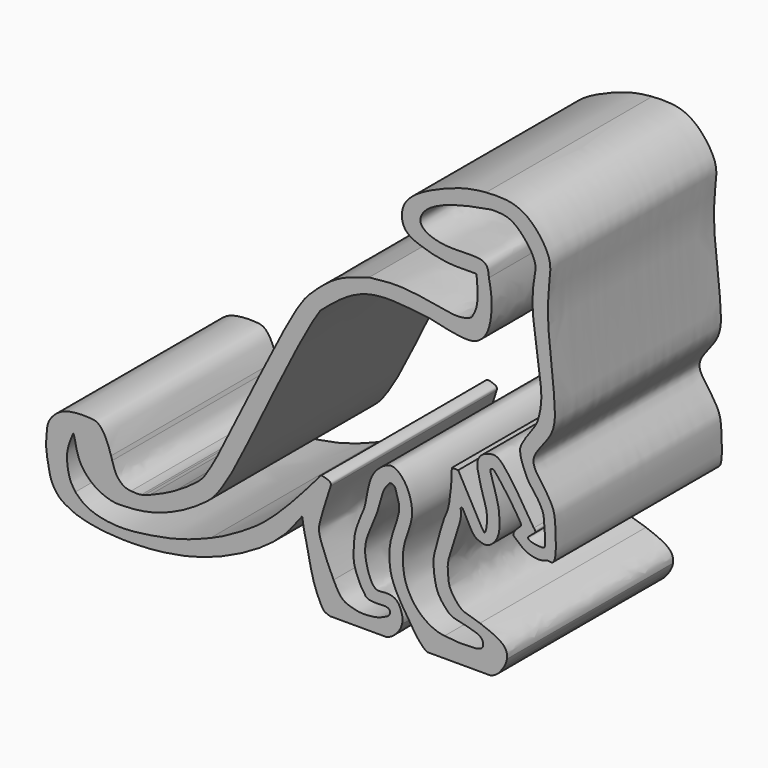
from build123d import *

# Parameters (mm, degrees)
F1_DEPTH = 15


with BuildPart() as f1:
    # F0 (on Front) → F1 (new body)
    with BuildSketch(Plane.XZ):
        with BuildLine():
            add(Edge.make_bspline(
                [(-15.4669350013, 23.1157913804), (-15.054879923, 23.1634013305), (-14.16984314, 23.2656608566), (-12.6167482466, 23.302404707), (-9.8137005936, 22.7928433269), (-8.9715752348, 22.6811060896), (-8.2451566536, 22.8389594973), (-8.03832151, 23.0131447315)],
                knots=[0, 0, 0, 0, 0.1348135249, 0.2895606307, 0.4912986818, 0.6066635572, 0.7214824154, 0.7214824154, 0.7214824154, 0.7214824154], degree=3))
            add(Edge.make_bspline(
                [(-15.4669350013, 23.1157913804), (-15.9986056397, 22.9585360257), (-17.0288350347, 22.6538187907), (-18.2910607324, 22.0040531604), (-19.6510649855, 20.7862506259), (-20.9749613494, 19.4248391371), (-26.1462638175, 8.5567205501), (-26.9967502917, 7.1942661965), (-27.6110490739, 6.1296289203), (-28.892969563, 5.3378997194), (-29.5255687088, 4.9558193423)],
                knots=[0, 0, 0, 0, 0.0832929576, 0.1614853434, 0.2445033573, 0.340585603, 0.5660088679, 0.6516770772, 0.7191066421, 0.8171798068, 0.8171798068, 0.8171798068, 0.8171798068], degree=3))
            add(Edge.make_bspline(
                [(-29.5255687088, 4.9558193423), (-30.0858358851, 4.6174263877), (-30.5959965363, 4.3182898855), (-31.2344844186, 4.148363515), (-31.2975818668, 4.1329435699)],
                knots=[0.8171798068, 0.8171798068, 0.8171798068, 0.8171798068, 0.9040391955, 0.9133811708, 0.9133811708, 0.9133811708, 0.9133811708], degree=3))
            add(Edge.make_bspline(
                [(-31.2975818668, 4.1329435699), (-31.4285690738, 4.083667204), (-31.5610759025, 4.0392471707), (-31.6864065826, 4.0075839497)],
                knots=[0.3472661829, 0.3472661829, 0.3472661829, 0.3472661829, 0.4123145482, 0.4123145482, 0.4123145482, 0.4123145482], degree=3))
            add(Edge.make_bspline(
                [(-31.9234459559, 3.935665863), (-31.8432725115, 3.9586455929), (-31.7648395471, 3.9831147713), (-31.6864065826, 4.0075839497)],
                knots=[0.9780776817, 0.9780776817, 0.9780776817, 0.9780776817, 1, 1, 1, 1], degree=3))
            add(Edge.make_bspline(
                [(-33.2431405897, 3.873629757), (-32.9938222307, 3.7955130583), (-32.4731148481, 3.7955338323), (-32.0677881033, 3.8942937655), (-31.9234459559, 3.935665863)],
                knots=[0.8714155003, 0.8714155003, 0.8714155003, 0.8714155003, 0.9386093201, 0.9780776817, 0.9780776817, 0.9780776817, 0.9780776817], degree=3))
            add(Edge.make_bspline(
                [(-38.7925319374, 5.3414250724), (-38.721084696, 5.9435743843), (-38.1788535617, 7.0706106992), (-36.3473578038, 7.4791844372), (-34.8143204132, 7.3092918194), (-34.2616133434, 5.6832398888), (-33.8553798627, 4.2615541077), (-33.4608473901, 3.9418418878), (-33.2431405897, 3.873629757)],
                knots=[0.3579762103, 0.3579762103, 0.3579762103, 0.3579762103, 0.452549549, 0.5488680078, 0.6332268885, 0.7246159405, 0.8127413153, 0.8714155003, 0.8714155003, 0.8714155003, 0.8714155003], degree=3))
            add(Edge.make_bspline(
                [(-36.6856083274, 1.167022041), (-36.9792061089, 1.3025797016), (-37.5137459028, 1.5493832146), (-37.995833183, 1.9429880165), (-38.4659027191, 2.6630431119), (-38.6351236587, 3.5813249337), (-38.8656756321, 4.7249782422), (-38.7925319374, 5.3414250724)],
                knots=[0, 0, 0, 0, 0.0692200048, 0.1260256358, 0.1907987089, 0.2611573089, 0.3579762103, 0.3579762103, 0.3579762103, 0.3579762103], degree=3))
            add(Edge.make_bspline(
                [(-33.264323081, 0.6425234606), (-33.956307962, 0.6583163529), (-35.3422405814, 0.7663689193), (-36.2294086305, 1.0309626238), (-36.6856083274, 1.167022041)],
                knots=[0.7985492923, 0.7985492923, 0.7985492923, 0.7985492923, 0.8964099847, 1, 1, 1, 1], degree=3))
            Line((-33.264323081, 0.6425234606), (-32.3675461113, 0.6425234606))
            add(Edge.make_bspline(
                [(-20.3062333167, 6.3436757773), (-20.6611693353, 5.8640278083), (-21.3773468926, 4.8962108139), (-22.7870587548, 3.6668792588), (-24.8786210821, 2.4010561969), (-27.3854524404, 1.3684346554), (-29.6188112156, 0.8474635726), (-31.3910469784, 0.6648604513), (-32.3675461113, 0.6425234606)],
                knots=[0, 0, 0, 0, 0.1111726523, 0.2243203123, 0.3548683181, 0.4919773448, 0.617850003, 0.756393634, 0.756393634, 0.756393634, 0.756393634], degree=3))
            add(Edge.make_bspline(
                [(-19.9869385811, 4.7234269858), (-20.0897746508, 5.2359042599), (-20.1980039837, 5.7897900186), (-20.3062333167, 6.3436757773)],
                knots=[0.8462860249, 0.8462860249, 0.8462860249, 0.8462860249, 1, 1, 1, 1], degree=3))
            add(Edge.make_bspline(
                [(-19.9869385811, 4.7234269858), (-19.8473422813, 4.2471836119), (-19.4359657855, 3.2454643685), (-18.6845972513, 1.5882668816), (-17.6524311989, 0.7718997519), (-16.4477854904, 0.6619995481), (-15.830565244, 0.6425234606)],
                knots=[0.0671721008, 0.0671721008, 0.0671721008, 0.0671721008, 0.1273073129, 0.1953228432, 0.2512897625, 0.3186434479, 0.3186434479, 0.3186434479, 0.3186434479], degree=3))
            Line((-15.830565244, 0.6425234606), (-15.1622339073, 0.6425234606))
            add(Edge.make_bspline(
                [(-15.1622339073, 0.6425234606), (-14.8462117896, 0.6556733045), (-14.1742418688, 0.7388745834), (-13.488866196, 1.1741118304), (-13.1493528322, 1.6241332052), (-13.083525002, 1.8462802982)],
                knots=[0.3437642472, 0.3437642472, 0.3437642472, 0.3437642472, 0.3809326547, 0.4292848272, 0.4727628742, 0.4727628742, 0.4727628742, 0.4727628742], degree=3))
            add(Edge.make_bspline(
                [(-13.083525002, 1.8462802982), (-13.0210016805, 2.0572757707), (-13.0702267264, 2.5242553153), (-13.4502605571, 3.3948452597), (-14.3400128819, 3.4715033442), (-15.0147359904, 3.3134605984), (-15.4314396869, 4.0176702238), (-15.6968701352, 4.8929884329), (-15.8753778927, 6.2254095225), (-14.9341280636, 8.0380593871), (-14.6419662461, 9.2001043005), (-14.4308895431, 9.9691338143), (-14.2066158173, 10.2474069961), (-14.1061712056, 10.3720361367)],
                knots=[0.4727628742, 0.4727628742, 0.4727628742, 0.4727628742, 0.5140583552, 0.5607435192, 0.606215053, 0.6457404287, 0.6875323254, 0.7359706555, 0.7934415444, 0.8650138478, 0.9208822959, 0.9645658579, 1, 1, 1, 1], degree=3))
            add(Edge.make_bspline(
                [(-14.1061712056, 10.3720361367), (-14.0759021809, 10.4147272319), (-14.0184900883, 10.4957006075), (-13.8973153211, 10.5385695894), (-13.7300823707, 10.5153843049), (-13.63781714, 10.4217180657), (-13.5888783261, 10.3720361367)],
                knots=[0, 0, 0, 0, 0.2450270904, 0.4647496284, 0.7160954557, 1, 1, 1, 1], degree=3))
            add(Edge.make_bspline(
                [(-13.5888783261, 10.3720361367), (-13.5120603733, 10.1381141839), (-13.3550850787, 9.6601013479), (-13.1961838953, 8.8573158626), (-13.9386883401, 7.0964644054), (-14.029511209, 5.8823634061), (-13.9312543069, 4.6407139263), (-13.3065154252, 3.3237249834), (-12.6931011566, 2.3996602204), (-12.3732164502, 1.9177767681)],
                knots=[0, 0, 0, 0, 0.1090299298, 0.2227995505, 0.3970254379, 0.5404619846, 0.6796758193, 0.8329565976, 1, 1, 1, 1], degree=3))
            add(Edge.make_bspline(
                [(-12.3732164502, 1.9177767681), (-12.222259227, 1.7001575863), (-11.9067441059, 1.2453125576), (-10.9894344382, 0.845283408), (-10.0343104079, 0.681105075), (-9.4010885805, 0.6425234606)],
                knots=[0, 0, 0, 0, 0.0932261165, 0.1948515535, 0.3298176717, 0.3298176717, 0.3298176717, 0.3298176717], degree=3))
            Line((-9.4010885805, 0.6425234606), (-8.0766113792, 0.6425234606))
            add(Edge.make_bspline(
                [(-8.0766113792, 0.6425234606), (-7.7567431744, 0.6622767608), (-6.9470527447, 0.75459554), (-6.2330828695, 1.0369075532), (-5.8991639222, 1.2783277634), (-5.7983550952, 1.3882837236)],
                knots=[0.4201952281, 0.4201952281, 0.4201952281, 0.4201952281, 0.4863778775, 0.595619114, 0.6586739236, 0.6586739236, 0.6586739236, 0.6586739236], degree=3))
            add(Edge.make_bspline(
                [(-5.4949996993, 2.0880033262), (-5.5148600395, 2.0058536231), (-5.5550412821, 1.8396491622), (-5.6629254997, 1.6083772376), (-5.7492481019, 1.4632361551), (-5.7983550952, 1.3882837236)],
                knots=[0, 0, 0, 0, 0.1495318737, 0.3025313974, 0.4362355704, 0.4362355704, 0.4362355704, 0.4362355704], degree=3))
            add(Edge.make_bspline(
                [(-5.4949996993, 2.0880033262), (-5.4701469369, 2.336698737), (-5.5925445679, 3.0257534011), (-6.7478403742, 3.4564712237), (-7.4563319795, 3.7206113338)],
                knots=[0.7604942681, 0.7604942681, 0.7604942681, 0.7604942681, 0.8531217723, 1, 1, 1, 1], degree=3))
            add(Edge.make_bspline(
                [(-7.4563319795, 3.7206113338), (-7.7590646166, 3.8040972055), (-8.2933435448, 3.9514375862), (-8.8073893838, 4.1496378846), (-9.1584104656, 4.5213102849), (-9.7439125381, 5.3180457664), (-9.7515011828, 6.2036080307), (-9.8739576405, 6.9715353464), (-8.8060644149, 9.6716500146), (-8.8227446636, 10.1987726152), (-8.8282274082, 10.3720361367)],
                knots=[0, 0, 0, 0, 0.1227682483, 0.2166680433, 0.3085905975, 0.4366305477, 0.5547268888, 0.6729520253, 0.8925003714, 1, 1, 1, 1], degree=3))
            add(Edge.make_bspline(
                [(-8.8282274082, 10.3720361367), (-8.8459191555, 10.4890795049), (-8.8735426347, 10.6718282753), (-8.7152589415, 10.6397863403), (-8.6191580919, 10.4609837355), (-7.9587578943, 9.1089874479), (-7.5537263871, 8.9515171078), (-7.0338059468, 8.7620230094), (-6.488104458, 9.0552033082), (-6.0060455478, 9.8002564148), (-6.0483343274, 10.9707100317), (-6.1263139378, 11.7653687297), (-6.5626727827, 13.1352722722), (-6.6911615079, 13.5359229006), (-6.7117596416, 13.8036617722), (-6.5443779215, 13.8213846123), (-6.3942248568, 13.8741403414), (-4.3728085734, 11.0126309837), (-4.5210199495, 10.8423260804), (-5.2176669074, 10.1787815682), (-4.8031479057, 9.9225054773), (-4.1561357097, 9.2342774925), (-2.9933199837, 9.0811120307), (-2.6148919685, 9.3663276273), (-1.8788251029, 9.0519584002), (-2.001532227, 11.7360439689), (-2.088144406, 12.6715776544), (-2.6466114232, 13.6253790471), (-3.2596811994, 14.4346665927), (-3.9401854687, 15.5886320501), (-2.0067838101, 17.3236857817), (-2.0171924895, 19.4292386241), (-2.3424064735, 22.3942466861), (-2.5630303766, 24.273281463), (-2.5516487553, 26.4525753793), (-2.2913474433, 27.931847581), (-2.5477930991, 29.0490720079), (-3.747573173, 30.6714568278), (-5.2732925212, 31.3601838866), (-6.4273675205, 31.3026820076), (-7.0113544352, 31.2735848129)],
                knots=[0, 0, 0, 0, 0.0139788176, 0.021826198, 0.0339469674, 0.0665891959, 0.0848900031, 0.1037653776, 0.1240039604, 0.1489816925, 0.1775217995, 0.2028273069, 0.2348160724, 0.2528158993, 0.265011323, 0.274361687, 0.2839657148, 0.3333905213, 0.3463682885, 0.3703502583, 0.3857999572, 0.4123526172, 0.4406737918, 0.4585459415, 0.4760313861, 0.5168043886, 0.5453992295, 0.5724650284, 0.6002514662, 0.6281950556, 0.6684683998, 0.7077081401, 0.7540592703, 0.7919902243, 0.8315598341, 0.8642430029, 0.8925560405, 0.9301648749, 0.964661916, 1, 1, 1, 1], degree=3))
            add(Edge.make_bspline(
                [(-7.7035482477, 25.8664894911), (-8.4457083434, 25.8407003297), (-9.9817336342, 25.8300480143), (-11.6753797268, 26.2960422118), (-13.138279716, 26.8972549511), (-13.2305676239, 29.0810860102), (-10.1990467685, 30.5339303208), (-8.2866784037, 31.146993755), (-7.3959278438, 31.2354113324), (-7.0113544352, 31.2735848129)],
                knots=[0.0496398748, 0.0496398748, 0.0496398748, 0.0496398748, 0.1744794615, 0.3161670076, 0.4346595673, 0.5636574426, 0.743202129, 0.8891298675, 1, 1, 1, 1], degree=3))
            add(Edge.make_bspline(
                [(-7.8565864766, 23.3494597612), (-7.7823789592, 23.5039601653), (-7.5550938606, 24.1069060212), (-7.6413982856, 25.1298405351), (-7.7035482477, 25.8664894911)],
                knots=[0.1755775827, 0.1755775827, 0.1755775827, 0.1755775827, 0.4062608835, 1, 1, 1, 1], degree=3))
            add(Edge.make_bspline(
                [(-8.03832151, 23.0131447315), (-7.9210122159, 23.1119361966), (-7.8537273009, 23.2414300938), (-7.8565864646, 23.3494597588)],
                knots=[0.7214824154, 0.7214824154, 0.7214824154, 0.7214824154, 0.7866034532, 0.7866034532, 0.7866034532, 0.7866034532], degree=3))
        make_face()
        with BuildLine():
            add(Edge.make_bspline(
                [(-9.6854204312, 21.6276198626), (-9.3858166443, 21.5767839844), (-8.7798707912, 21.473968897), (-7.7486266166, 21.4238348023), (-6.725168976, 22.3308861229), (-6.5241565721, 24.5201787013), (-6.7220458497, 25.4745487116), (-6.8110576831, 25.9038303047)],
                knots=[0, 0, 0, 0, 0.1686051123, 0.3410022606, 0.5344340169, 0.7905855121, 1, 1, 1, 1], degree=3))
            add(Edge.make_bspline(
                [(-6.6328905523, 30.2999410778), (-6.9912906796, 30.2393266557), (-7.7957819357, 30.1017143669), (-9.6311830725, 29.6926698718), (-11.4767502972, 28.8938746516), (-12.0662389547, 27.5094989035), (-9.8203611908, 26.6698072252), (-6.9183895832, 27.1949228854), (-6.8410419305, 26.2706124885), (-6.8110576831, 25.9038303047)],
                knots=[0, 0, 0, 0, 0.1200716158, 0.275554394, 0.4347600187, 0.547090701, 0.7074931298, 0.8911373827, 1, 1, 1, 1], degree=3))
            add(Edge.make_bspline(
                [(-3.0616135336, 20.267073065), (-3.2686607835, 21.7765539786), (-3.5891472989, 24.113065467), (-3.6913634177, 25.2814257531), (-3.6017700921, 26.8324184474), (-3.3224314813, 27.7894600366), (-3.8556647148, 28.817991088), (-4.6577014721, 29.7562568509), (-5.4976916544, 30.3002019753), (-6.2450947406, 30.3000302031), (-6.6328905523, 30.2999410778)],
                knots=[0, 0, 0, 0, 0.2097043255, 0.324599378, 0.4530649063, 0.5572912366, 0.667233028, 0.7851825486, 0.8885403212, 1, 1, 1, 1], degree=3))
            add(Edge.make_bspline(
                [(-3.5657018889, 11.042711325), (-3.502401173, 10.9800372772), (-3.340229767, 10.8194713449), (-3.8677361259, 10.4617169154), (-4.0239852675, 10.2877857668), (-3.885334559, 10.1256749549), (-3.4480939544, 10.0118742901), (-2.834917621, 9.9799016557), (-2.7203748773, 10.1748078404), (-2.7945969032, 11.7444956991), (-2.9106171164, 12.4318540116), (-3.5684221248, 13.418532929), (-3.9774941234, 13.8259430343), (-4.4601771998, 15.0091519055), (-4.5496488595, 15.4863993988), (-4.5928707234, 16.0286914779), (-3.6357387515, 17.2950574509), (-3.2618118711, 17.8625227488), (-2.9692878273, 19.2245714238), (-3.0319232899, 19.9318237711), (-3.0616135336, 20.267073065)],
                knots=[0, 0, 0, 0, 0.032618196, 0.0835652272, 0.1146446208, 0.1408854115, 0.1879268674, 0.2395625518, 0.2675202674, 0.350704353, 0.4126961873, 0.4832652047, 0.5379249416, 0.6132710084, 0.6607985958, 0.7086665933, 0.7924530461, 0.8517218511, 0.9297137084, 1, 1, 1, 1], degree=3))
            add(Edge.make_bspline(
                [(-9.0274596587, 12.9462070763), (-8.2591746595, 11.5188340752), (-7.3345520081, 9.8010061727), (-7.0892435421, 9.5189452518), (-6.9355623846, 10.0833829326), (-6.9322018719, 11.0260947431), (-7.2176893727, 11.7814879305), (-7.5936640744, 13.198009107), (-7.7169242278, 14.0269100902), (-7.2796674947, 14.5865419851), (-6.5971197275, 14.7803430515), (-5.8354696532, 14.7237171829), (-4.5261455694, 12.6003150895), (-3.5657018889, 11.042711325)],
                knots=[0, 0, 0, 0, 0.1683925456, 0.2026585996, 0.2607106631, 0.3466726556, 0.4269436174, 0.5326912861, 0.6115565667, 0.6806686762, 0.7517072843, 0.8178669646, 1, 1, 1, 1], degree=3))
            add(Edge.make_bspline(
                [(-9.489021264, 12.9462070763), (-9.3351673956, 12.9462070763), (-9.1813135271, 12.9462070763), (-9.0274596587, 12.9462070763)],
                knots=[0, 0, 0, 0, 0.4615616053, 0.4615616053, 0.4615616053, 0.4615616053], degree=3))
            add(Edge.make_bspline(
                [(-9.736799635, 3.6653678399), (-9.955313621, 3.8779464445), (-10.3120224644, 4.294094476), (-10.7038451024, 5.0484805445), (-10.8683131809, 6.6471407267), (-10.7018549207, 7.25561029), (-10.1030872824, 9.5469927127), (-9.7587928827, 10.1127232644), (-9.5317904183, 11.4541108734), (-9.5037597065, 12.4320240283), (-9.489021264, 12.9462070763)],
                knots=[0.2531916343, 0.2531916343, 0.2531916343, 0.2531916343, 0.3319345472, 0.4123423186, 0.5178848032, 0.5928006938, 0.7220552944, 0.7960207863, 0.8927484989, 1, 1, 1, 1], degree=3))
            add(Edge.make_bspline(
                [(-9.736799635, 3.6653678399), (-9.6680512117, 3.6087654322), (-9.5091615974, 3.4779473814), (-9.0320435402, 3.3632203663), (-8.4460986817, 3.2350185077), (-7.9281081042, 3.0922920026), (-7.492030474, 2.9495224622), (-7.219005629, 2.6671015653), (-7.2077523949, 2.2520788072), (-7.4806210356, 2.0480485861), (-8.0419411238, 1.9949798277), (-9.061641678, 1.9643852309), (-9.6990536772, 2.0437683351), (-10.0131081417, 2.0828805864)],
                knots=[0, 0, 0, 0, 0.0669612444, 0.1547591317, 0.2540428249, 0.3474352007, 0.4322426786, 0.5090920239, 0.585212863, 0.6531411917, 0.7467128933, 0.8752048176, 1, 1, 1, 1], degree=3))
            add(Edge.make_bspline(
                [(-15.7243199646, 2.7652664576), (-15.8215515456, 2.90688523), (-16.0569856631, 3.2368973641), (-16.2985209482, 3.7810798689), (-16.6242987526, 4.6077361362), (-16.5754242127, 5.5606333607), (-16.5534606755, 6.4673363388), (-16.1127968214, 7.670513616), (-15.7314510826, 8.3898188184), (-15.5487725157, 9.9048338682), (-15.0993902808, 11.0072168655), (-14.0156723105, 11.7782557779), (-13.3412969058, 11.5046842592), (-12.6742022677, 10.7273450001), (-12.3210082887, 9.5290593405), (-12.3735580544, 8.5597871155), (-12.8438481056, 7.3540611631), (-13.0781965424, 6.3486107107), (-12.9813116625, 4.7911242558), (-12.453041769, 3.707239257), (-11.821605295, 2.8905006169), (-10.8615763932, 2.2476983817), (-10.2819966319, 2.1133552685), (-10.0131081417, 2.0828805864)],
                knots=[0.0794669175, 0.0794669175, 0.0794669175, 0.0794669175, 0.108239044, 0.1381150811, 0.1740469277, 0.2112951767, 0.2483867237, 0.2910555429, 0.3263955273, 0.3730077291, 0.4158324242, 0.4575304018, 0.4877998864, 0.5261795019, 0.5687669007, 0.6067088802, 0.6496814325, 0.6893163433, 0.7366998088, 0.7788291018, 0.8177163353, 0.8585709235, 0.893993386, 0.893993386, 0.893993386, 0.893993386], degree=3))
            add(Edge.make_bspline(
                [(-15.7243199646, 2.7652664576), (-15.6881908943, 2.7240265419), (-15.5962218717, 2.6190475127), (-15.149286357, 2.5524278186), (-14.6994437069, 2.5623149844), (-14.136083725, 2.6024548929), (-13.9054191571, 2.375230356), (-14.0073176849, 2.0436123106), (-14.3264996419, 1.8905074485), (-14.8953565292, 1.6240174721), (-15.8713943909, 1.5585383986), (-16.3224319706, 1.5987435197), (-16.9150557322, 1.759736622), (-17.2959177098, 1.9125323799), (-17.6840808041, 2.3230153053), (-17.9092213718, 2.7822345224), (-18.033541739, 3.0358107761)],
                knots=[0, 0, 0, 0, 0.0436894939, 0.1112145983, 0.1840013853, 0.260440224, 0.3132964026, 0.3687172059, 0.428394401, 0.5114901109, 0.6133846972, 0.6850643674, 0.7645399488, 0.8308055071, 0.9065724951, 1, 1, 1, 1], degree=3))
            add(Edge.make_bspline(
                [(-18.2472337037, 8.9346179739), (-18.283626976, 8.8074305111), (-18.3741080033, 8.4912167838), (-18.6846136933, 7.6074015726), (-19.0400290014, 6.3790763296), (-19.1595046681, 5.688373645), (-18.5823015223, 4.2473625461), (-18.2453439829, 3.4322379405), (-18.033541739, 3.0358107761)],
                knots=[0, 0, 0, 0, 0.0620932169, 0.1543762815, 0.2608754986, 0.3394483968, 0.4540893616, 0.5649108011, 0.5649108011, 0.5649108011, 0.5649108011], degree=3))
            add(Edge.make_bspline(
                [(-19.1535390913, 9.1417562217), (-19.0920071207, 9.2377298206), (-18.9685999394, 9.4302123822), (-18.6461759477, 9.3464596063), (-18.1908161646, 9.1864113862), (-18.2308653417, 9.007670535), (-18.2472337037, 8.9346179739)],
                knots=[0, 0, 0, 0, 0.2486531754, 0.4986933978, 0.7951126956, 1, 1, 1, 1], degree=3))
            add(Edge.make_bspline(
                [(-26.9343461841, 2.8049554676), (-26.3844964414, 3.0177295796), (-25.2203599978, 3.6379405454), (-23.1404632208, 4.8810752251), (-21.0081338928, 6.9958170821), (-19.7662589823, 8.4327821673), (-19.1535390913, 9.1417562217)],
                knots=[0.4315646956, 0.4315646956, 0.4315646956, 0.4315646956, 0.5538581506, 0.6933479209, 0.8487030965, 1, 1, 1, 1], degree=3))
            add(Edge.make_bspline(
                [(-36.6939082742, 2.5590115692), (-36.4601219719, 2.3190888141), (-35.8981242558, 1.7423397099), (-33.7494408389, 1.2352257638), (-31.3307350271, 1.5391222372), (-29.0668777687, 1.9565132815), (-27.6443911487, 2.5224592521), (-26.9343461841, 2.8049554676)],
                knots=[0, 0, 0, 0, 0.1458891159, 0.3507021119, 0.5732130235, 0.7869660499, 1, 1, 1, 1], degree=3))
            add(Edge.make_bspline(
                [(-36.6939082742, 2.5590115692), (-36.80788912, 2.7228948404), (-37.0526104297, 3.0747585985), (-37.2714345607, 3.8591197057), (-37.3649904858, 5.0638266879), (-37.0139818985, 5.8609988534), (-36.833640188, 6.2705711462)],
                knots=[0, 0, 0, 0, 0.1995096526, 0.4283549848, 0.7062993797, 1, 1, 1, 1], degree=3))
            Line((-36.833640188, 6.2705711462), (-36.7119126022, 5.7930187322))
            add(Edge.make_bspline(
                [(-32.4920768623, 2.839992533), (-32.7180122089, 2.817175661), (-33.3349776724, 2.7739393621), (-34.0468326401, 2.7883544929), (-35.1945453707, 3.2026078031), (-36.2058608103, 4.1423555444), (-36.5816519473, 5.1045443733), (-36.6714243479, 5.5790237625), (-36.7119126022, 5.7930187322)],
                knots=[0.3566105639, 0.3566105639, 0.3566105639, 0.3566105639, 0.4156439103, 0.5273366541, 0.6525891868, 0.7881356198, 0.9044470367, 1, 1, 1, 1], degree=3))
            add(Edge.make_bspline(
                [(-32.6518937945, 2.9238865245), (-32.598951013, 2.8958555106), (-32.5460082315, 2.8678244967), (-32.4920768627, 2.8399925326)],
                knots=[0, 0, 0, 0, 0.0184438751, 0.0184438751, 0.0184438751, 0.0184438751], degree=3))
            add(Edge.make_bspline(
                [(-31.0687634358, 3.0878764336), (-31.5790931903, 2.9915283861), (-32.1154934924, 2.9577074553), (-32.6518937945, 2.9238865245)],
                knots=[0.9198628773, 0.9198628773, 0.9198628773, 0.9198628773, 1, 1, 1, 1], degree=3))
            add(Edge.make_bspline(
                [(-28.9265941828, 3.9377333596), (-29.1854313038, 3.8083492808), (-29.7358238202, 3.5332263445), (-30.5811984483, 3.2166498449), (-31.0687634358, 3.0878764336)],
                knots=[0, 0, 0, 0, 0.1116713141, 0.237458427, 0.237458427, 0.237458427, 0.237458427], degree=3))
            add(Edge.make_bspline(
                [(-18.9958438277, 19.8572631925), (-20.3235491735, 17.9981015241), (-24.9123949819, 8.0944324706), (-26.0372922996, 6.3969000052), (-26.8555018394, 5.1674900195), (-28.2225464252, 4.3263449115), (-28.9265941828, 3.9377333596)],
                knots=[0.2550488056, 0.2550488056, 0.2550488056, 0.2550488056, 0.508599348, 0.6154355514, 0.6947226707, 0.8038378277, 0.8038378277, 0.8038378277, 0.8038378277], degree=3))
            add(Edge.make_bspline(
                [(-9.6854204312, 21.6276198626), (-10.0972466375, 21.7295887974), (-10.974654365, 21.9468365829), (-12.6084409295, 22.1130910967), (-15.033478598, 22.3103972254), (-17.1339446237, 21.466571727), (-18.364731646, 20.4027568573), (-18.9958438277, 19.8572631925)],
                knots=[0, 0, 0, 0, 0.1618551998, 0.3448372175, 0.5652744113, 0.7770852229, 1, 1, 1, 1], degree=3))
        make_face(mode=Mode.SUBTRACT)
        with BuildLine():
            add(Edge.make_bspline(
                [(-29.5255687088, 4.9558193423), (-30.0858358851, 4.6174263877), (-30.5959965363, 4.3182898855), (-31.2344844186, 4.148363515), (-31.2975818668, 4.1329435699)],
                knots=[0.8171798068, 0.8171798068, 0.8171798068, 0.8171798068, 0.9040391955, 0.9133811708, 0.9133811708, 0.9133811708, 0.9133811708], degree=3))
            add(Edge.make_bspline(
                [(-29.5255687088, 4.9558193423), (-29.7746350144, 4.8285893471), (-30.2453715043, 4.5786059943), (-30.7137648316, 4.375294171), (-31.1259868263, 4.1974962863), (-31.2975818668, 4.1329435699)],
                knots=[0, 0, 0, 0, 0.1393972042, 0.2620519308, 0.3472661829, 0.3472661829, 0.3472661829, 0.3472661829], degree=3))
        make_face()
        with BuildLine():
            add(Edge.make_bspline(
                [(-8.03832151, 23.0131447315), (-7.9756947149, 23.1225057178), (-7.9130672728, 23.2318664747), (-7.8565864766, 23.3494597612)],
                knots=[0, 0, 0, 0, 0.1755775827, 0.1755775827, 0.1755775827, 0.1755775827], degree=3))
            add(Edge.make_bspline(
                [(-8.03832151, 23.0131447315), (-7.9210122159, 23.1119361966), (-7.8537273009, 23.2414300938), (-7.8565864646, 23.3494597588)],
                knots=[0.7214824154, 0.7214824154, 0.7214824154, 0.7214824154, 0.7866034532, 0.7866034532, 0.7866034532, 0.7866034532], degree=3))
        make_face()
        with BuildLine():
            add(Edge.make_bspline(
                [(-32.6745203681, 3.9277919449), (-32.5832057085, 3.9170489794), (-32.3574760456, 3.9019853255), (-32.101904133, 3.906913157), (-31.977228499, 3.9261791625), (-31.9386237804, 3.9326100183), (-31.9234459559, 3.935665863)],
                knots=[0.7168111336, 0.7168111336, 0.7168111336, 0.7168111336, 0.7898228616, 0.8944951802, 0.9581950641, 1, 1, 1, 1], degree=3))
            add(Edge.make_bspline(
                [(-32.6745203681, 3.9277919449), (-32.8625520871, 3.9094227995), (-33.0527605765, 3.8921633959), (-33.2431405897, 3.873629757)],
                knots=[0.9757976067, 0.9757976067, 0.9757976067, 0.9757976067, 1, 1, 1, 1], degree=3))
            add(Edge.make_bspline(
                [(-33.2431405897, 3.873629757), (-32.9938222307, 3.7955130583), (-32.4731148481, 3.7955338323), (-32.0677881033, 3.8942937655), (-31.9234459559, 3.935665863)],
                knots=[0.8714155003, 0.8714155003, 0.8714155003, 0.8714155003, 0.9386093201, 0.9780776817, 0.9780776817, 0.9780776817, 0.9780776817], degree=3))
        make_face()
        with BuildLine():
            add(Edge.make_bspline(
                [(-32.6745203681, 3.9277919449), (-32.8625520871, 3.9094227995), (-33.0527605765, 3.8921633959), (-33.2431405897, 3.873629757)],
                knots=[0.9757976067, 0.9757976067, 0.9757976067, 0.9757976067, 1, 1, 1, 1], degree=3))
            add(Edge.make_bspline(
                [(-34.0348669257, 5.4219118734), (-33.9768485678, 5.2298243481), (-33.8596540727, 4.8647910229), (-33.6969160928, 4.5448480297), (-33.5936358249, 4.4225677588), (-33.3886925788, 4.2074026246), (-33.2052466634, 4.0621846525), (-32.9477243451, 3.9680562646), (-32.7441083533, 3.9359788157), (-32.6745203681, 3.9277919449)],
                knots=[0.0550801718, 0.0550801718, 0.0550801718, 0.0550801718, 0.1713008915, 0.2878121757, 0.3617973174, 0.4612562915, 0.5520281007, 0.6611712279, 0.7168111336, 0.7168111336, 0.7168111336, 0.7168111336], degree=3))
            add(Edge.make_bspline(
                [(-34.0348669257, 5.4219118734), (-33.9551196544, 5.1473706732), (-33.817565169, 4.6605504497), (-33.5947869935, 4.2828724777), (-33.474297277, 4.0439580542), (-33.3215633687, 3.9314157487), (-33.2431405897, 3.873629757)],
                knots=[0.7758670544, 0.7758670544, 0.7758670544, 0.7758670544, 0.8453793037, 0.9071218112, 0.9523107491, 1, 1, 1, 1], degree=3))
        make_face()
        with BuildLine():
            add(Edge.make_bspline(
                [(-38.7925319374, 5.3414250724), (-38.721084696, 5.9435743843), (-38.1788535617, 7.0706106992), (-36.3473578038, 7.4791844372), (-34.8143204132, 7.3092918194), (-34.2616133434, 5.6832398888), (-33.8553798627, 4.2615541077), (-33.4608473901, 3.9418418878), (-33.2431405897, 3.873629757)],
                knots=[0.3579762103, 0.3579762103, 0.3579762103, 0.3579762103, 0.452549549, 0.5488680078, 0.6332268885, 0.7246159405, 0.8127413153, 0.8714155003, 0.8714155003, 0.8714155003, 0.8714155003], degree=3))
            add(Edge.make_bspline(
                [(-34.0348669257, 5.4219118734), (-33.9551196544, 5.1473706732), (-33.817565169, 4.6605504497), (-33.5947869935, 4.2828724777), (-33.474297277, 4.0439580542), (-33.3215633687, 3.9314157487), (-33.2431405897, 3.873629757)],
                knots=[0.7758670544, 0.7758670544, 0.7758670544, 0.7758670544, 0.8453793037, 0.9071218112, 0.9523107491, 1, 1, 1, 1], degree=3))
            add(Edge.make_bspline(
                [(-34.1171287, 5.6994184852), (-34.0897463022, 5.6061837826), (-34.0623634094, 5.5129473955), (-34.0348669257, 5.4219118734)],
                knots=[0, 0, 0, 0, 0.0550801718, 0.0550801718, 0.0550801718, 0.0550801718], degree=3))
            add(Edge.make_bspline(
                [(-38.7925319374, 5.3414250724), (-38.7775971357, 5.615663083), (-38.7507807918, 6.108074093), (-38.5664698086, 6.5769736079), (-38.1925599317, 7.0289940014), (-37.659812499, 7.3977120776), (-37.029428279, 7.5725317804), (-36.2520816561, 7.6383412475), (-35.7051146118, 7.6159753607), (-35.0628527943, 7.580124938), (-34.5135525689, 6.8600118416), (-34.2418872275, 6.1074280456), (-34.1171287, 5.6994184852)],
                knots=[0, 0, 0, 0, 0.0790917663, 0.1420140718, 0.2099411256, 0.281733448, 0.354806913, 0.4338715773, 0.5010922365, 0.5696313926, 0.6518993466, 0.7527860975, 0.7527860975, 0.7527860975, 0.7527860975], degree=3))
        make_face()
        with BuildLine():
            add(Edge.make_bspline(
                [(-31.0687634358, 3.0878764336), (-31.1589515879, 3.0640563557), (-31.6277637956, 2.9488957474), (-32.1251031305, 2.8770526602), (-32.4920768623, 2.839992533)],
                knots=[0.237458427, 0.237458427, 0.237458427, 0.237458427, 0.2607261094, 0.3566105639, 0.3566105639, 0.3566105639, 0.3566105639], degree=3))
            add(Edge.make_bspline(
                [(-31.0687634358, 3.0878764336), (-31.5790931903, 2.9915283861), (-32.1154934924, 2.9577074553), (-32.6518937945, 2.9238865245)],
                knots=[0.9198628773, 0.9198628773, 0.9198628773, 0.9198628773, 1, 1, 1, 1], degree=3))
            add(Edge.make_bspline(
                [(-32.6518937945, 2.9238865245), (-32.598951013, 2.8958555106), (-32.5460082315, 2.8678244967), (-32.4920768627, 2.8399925326)],
                knots=[0, 0, 0, 0, 0.0184438751, 0.0184438751, 0.0184438751, 0.0184438751], degree=3))
        make_face()
        with BuildLine():
            add(Edge.make_bspline(
                [(-5.7983550952, 1.3882837236), (-5.8102442807, 1.3701371564), (-5.8993347281, 1.2367849642), (-6.1045058924, 0.9599609252), (-6.3582924798, 0.7828342894), (-6.5484015026, 0.6893370734), (-6.643588189, 0.6425234606)],
                knots=[0.4362355704, 0.4362355704, 0.4362355704, 0.4362355704, 0.4686063918, 0.6686613218, 0.8341002946, 1, 1, 1, 1], degree=3))
            add(Edge.make_bspline(
                [(-8.0766113792, 0.6425234606), (-7.7567431744, 0.6622767608), (-6.9470527447, 0.75459554), (-6.2330828695, 1.0369075532), (-5.8991639222, 1.2783277634), (-5.7983550952, 1.3882837236)],
                knots=[0.4201952281, 0.4201952281, 0.4201952281, 0.4201952281, 0.4863778775, 0.595619114, 0.6586739236, 0.6586739236, 0.6586739236, 0.6586739236], degree=3))
            Line((-8.0766113792, 0.6425234606), (-6.643588189, 0.6425234606))
        make_face()
        with BuildLine():
            add(Edge.make_bspline(
                [(-18.2802025229, 0.6425234606), (-18.3946654866, 0.6770942934), (-18.618768649, 0.7447793569), (-18.8734558337, 0.9515868547), (-19.3418080442, 2.0262211595), (-19.5854957246, 2.7778101959), (-19.8430831598, 4.006532278), (-19.9869385811, 4.7234269858)],
                knots=[0, 0, 0, 0, 0.1150647556, 0.2252813904, 0.430773902, 0.6312584699, 0.8462860249, 0.8462860249, 0.8462860249, 0.8462860249], degree=3))
            Line((-18.2802025229, 0.6425234606), (-15.830565244, 0.6425234606))
            add(Edge.make_bspline(
                [(-19.9869385811, 4.7234269858), (-19.8473422813, 4.2471836119), (-19.4359657855, 3.2454643685), (-18.6845972513, 1.5882668816), (-17.6524311989, 0.7718997519), (-16.4477854904, 0.6619995481), (-15.830565244, 0.6425234606)],
                knots=[0.0671721008, 0.0671721008, 0.0671721008, 0.0671721008, 0.1273073129, 0.1953228432, 0.2512897625, 0.3186434479, 0.3186434479, 0.3186434479, 0.3186434479], degree=3))
        make_face()
        with BuildLine():
            add(Edge.make_bspline(
                [(-19.9869385811, 4.7234269858), (-20.0897746508, 5.2359042599), (-20.1980039837, 5.7897900186), (-20.3062333167, 6.3436757773)],
                knots=[0.8462860249, 0.8462860249, 0.8462860249, 0.8462860249, 1, 1, 1, 1], degree=3))
            add(Edge.make_bspline(
                [(-20.3062333167, 6.3436757773), (-20.2308201286, 5.8393574151), (-20.1494270957, 5.2950494225), (-19.9983946777, 4.7625103292), (-19.9869385811, 4.7234269858)],
                knots=[0, 0, 0, 0, 0.0622370502, 0.0671721008, 0.0671721008, 0.0671721008, 0.0671721008], degree=3))
        make_face()
        with BuildLine():
            Line((-11.2530905753, 0.6425234606), (-9.4010885805, 0.6425234606))
            add(Edge.make_bspline(
                [(-12.3732164502, 1.9177767681), (-12.222259227, 1.7001575863), (-11.9067441059, 1.2453125576), (-10.9894344382, 0.845283408), (-10.0343104079, 0.681105075), (-9.4010885805, 0.6425234606)],
                knots=[0, 0, 0, 0, 0.0932261165, 0.1948515535, 0.3298176717, 0.3298176717, 0.3298176717, 0.3298176717], degree=3))
            add(Edge.make_bspline(
                [(-11.2530905753, 0.6425234606), (-11.3129005804, 0.6735439933), (-11.460075734, 0.749876568), (-11.7873613246, 1.08065143), (-12.1827324294, 1.571809119), (-12.3152735481, 1.8125376538), (-12.3732164502, 1.9177767681)],
                knots=[0, 0, 0, 0, 0.1814180555, 0.4464174541, 0.7579907306, 1, 1, 1, 1], degree=3))
        make_face()
        with BuildLine():
            add(Edge.make_bspline(
                [(-15.1622339073, 0.6425234606), (-14.8462117896, 0.6556733045), (-14.1742418688, 0.7388745834), (-13.488866196, 1.1741118304), (-13.1493528322, 1.6241332052), (-13.083525002, 1.8462802982)],
                knots=[0.3437642472, 0.3437642472, 0.3437642472, 0.3437642472, 0.3809326547, 0.4292848272, 0.4727628742, 0.4727628742, 0.4727628742, 0.4727628742], degree=3))
            Line((-15.1622339073, 0.6425234606), (-14.188233763, 0.6425234606))
            add(Edge.make_bspline(
                [(-13.083525002, 1.8462802982), (-13.1166266358, 1.7317971626), (-13.1892910411, 1.4804848251), (-13.5218891996, 1.0521599898), (-13.8349357698, 0.7817856127), (-14.0727118276, 0.6880596189), (-14.188233763, 0.6425234606)],
                knots=[0, 0, 0, 0, 0.23571649, 0.5174426936, 0.7655527032, 1, 1, 1, 1], degree=3))
        make_face()
    extrude(amount=F1_DEPTH)


solid = f1.part
